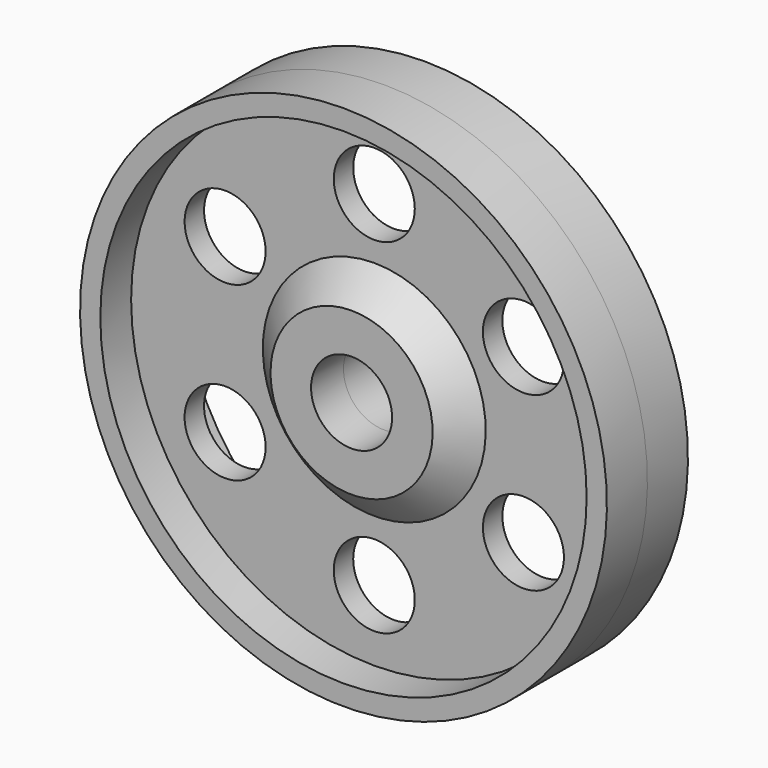
from build123d import *

# Parameters (mm, degrees)
F5_R            = 20
F6_DEPTH        = 25
F6_COPIES_COUNT = 6


# Not quite as in the source:
# - a pattern or mirror of a feature is missing from the dataset's text; its kind, count and spacing are read off the source's solid


with BuildPart() as f3:
    # F0 (on Right) → F3 (revolve)
    with BuildSketch(Plane.YZ):
        Polygon((25, 130), (0, 130), (0, 20), (20, 20), (20, 40), (6, 55), (6, 120), (25, 120), align=None)
    revolve(axis=Axis((0, 0.1935698092, 0), (0, -1, 0)))

    # F4: F3 across plane


with BuildPart() as f3_1:
    add(f3.part)
    add(f3.part.mirror(Plane.XZ))

    # F5 (on face) → F6 (cut)
    with BuildSketch(Plane.XZ.offset(6)):
        with Locations((0, 85)):
            Circle(F5_R)
    f6 = extrude(amount=-F6_DEPTH, mode=Mode.SUBTRACT)

    # F6_copies: F6 ×6 about axis
    f6_copies_axis = Axis((0, 0, 0), (0, 1, 0))
    for i in range(1, F6_COPIES_COUNT):
        add(f6.rotate(f6_copies_axis, i * 360 / F6_COPIES_COUNT), mode=Mode.SUBTRACT)


solid = f3_1.part
